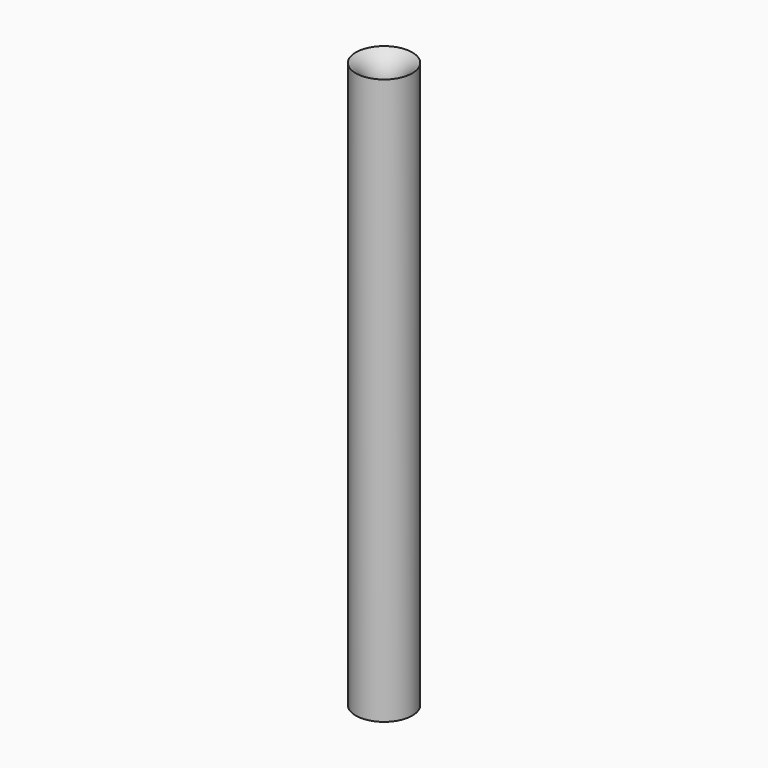
from build123d import *

# Parameters (mm, degrees)
F0_R     = 5
F0_R_2   = 2.5
F1_DEPTH = 100


# Not quite as in the source:
# - a fillet or chamfer that OpenCascade refuses, or shapes differently, is made with other operations: its cross-section is extruded or revolved along the edge and cut away or added


with BuildPart() as f1:
    # F0 (on Top) → F1 (new body)
    with BuildSketch(Plane.XY):
        Circle(F0_R)
        Circle(F0_R_2, mode=Mode.SUBTRACT)
    extrude(amount=F1_DEPTH)

    # F2: fillet of radius 5 on 1 edges, made by hand

    # F2_s1 → F2_t2 (revolve, cut)
    with BuildSketch(Plane.XZ):
        with BuildLine():
            ThreePointArc((2.5, 95.6698729811), (3.1698729811, 98.1698729811), (5, 100))
            Line((5, 100), (2.5, 100))
            Line((2.5, 100), (2.5, 95.6698729811))
        make_face()
    revolve(axis=Axis((0, 0, 100), (0, 0, 1)), mode=Mode.SUBTRACT)

    # F3: fillet of radius 5 on 1 edges, made by hand

    # F3_s1 → F3_t2 (revolve, cut)
    with BuildSketch(Plane.XZ):
        with BuildLine():
            ThreePointArc((5, 0), (3.1698729811, 1.8301270189), (2.5, 4.3301270189))
            Line((2.5, 4.3301270189), (2.5, 0))
            Line((2.5, 0), (5, 0))
        make_face()
    revolve(axis=Axis((0, 0, 0), (0, 0, 1)), mode=Mode.SUBTRACT)


solid = f1.part
